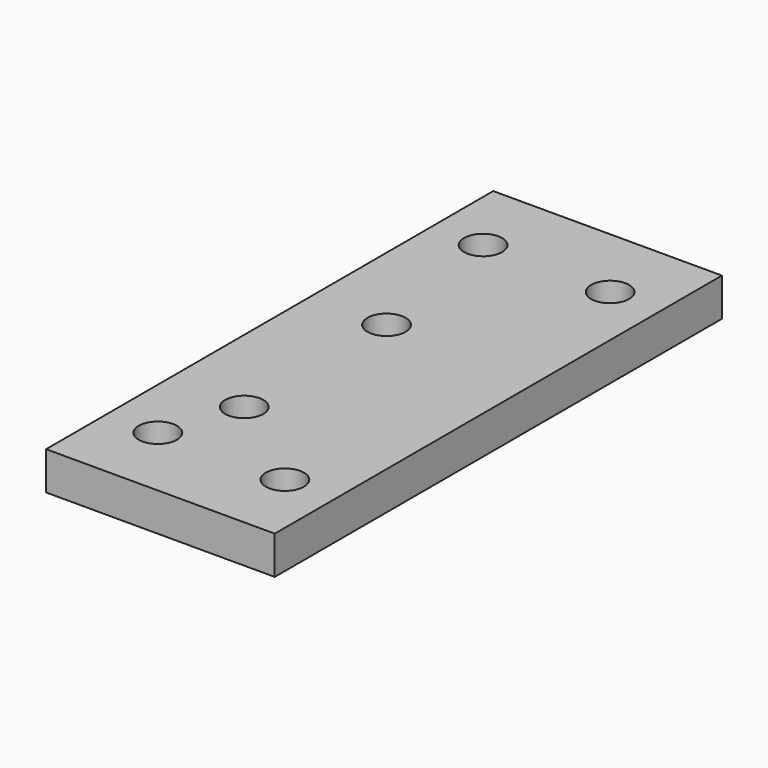
from build123d import *

# Parameters (mm, degrees)
F0_W     = 18
F0_H     = 44
F1_DEPTH = 3
F2_D     = 3


# Not quite as in the source:
# - a feature names something its author has since deleted; it is built from what else it names


with BuildPart() as f1:
    # F0 (on Top) → F1 (new body)
    with BuildSketch(Plane.XY):
        Rectangle(F0_W, F0_H)
    extrude(amount=F1_DEPTH)

    # F2 (through all)
    with Locations(Plane(origin=(0, 0, 0), x_dir=(1, 0, 0), z_dir=(0, 0, -1))):
        with Locations((-5, -16), (5, 16), (5, -16), (-5, 16), (-3, 10), (-3, -4)):
            Hole(F2_D / 2)


solid = f1.part
